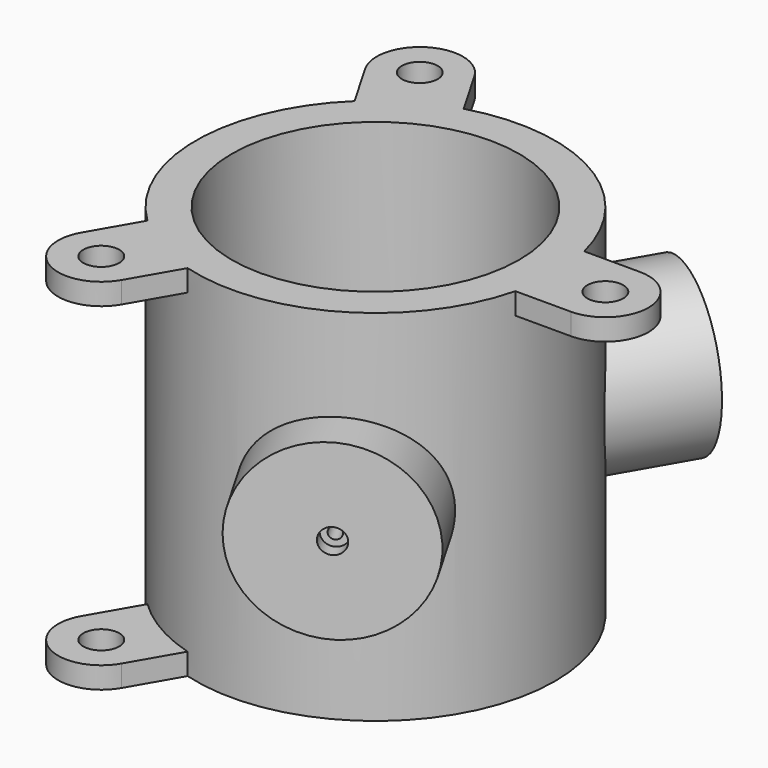
from build123d import *

# Parameters (mm, degrees)
F1_R             = 125
F1_R_2           = 100
F2_DEPTH         = 250
F3_R             = 12.5
F4_DEPTH         = 15
F4_COPIES_COUNT  = 3
F4_COPIES1_COUNT = 2
F10_R            = 56.8493867215
F10_R_2          = 5
F10_R_3          = 28.1619206838
F11_DEPTH        = 68.6754869442
F15_R            = 60.4503373428
F18_D            = 8.5
F18_CBORE_D      = 17.25
F18_CBORE_DEPTH  = 10


# Not quite as in the source:
# - ends of sketch curves that miss each other by under 0.0002 mm in the source are joined
# - a pattern or mirror of a feature is missing from the dataset's text; its kind, count and spacing are read off the source's solid


with BuildPart() as f2:
    # F1 (on offset) → F2 (new body)
    with BuildSketch(Plane.XY.offset(125)):
        Circle(F1_R)
        Circle(F1_R_2, mode=Mode.SUBTRACT)
    extrude(amount=-F2_DEPTH)

    # F3 (on face) → F4 (join)
    with BuildSketch(Plane.XY.offset(125)):
        with BuildLine():
            Line((-105.9807621135, 123.5640646055), (-86.6540676111, 90.0892477849))
            ThreePointArc((-86.6540676111, 90.0892477849), (-62.5, 108.2531754731), (-34.692543384, 120.0892477849))
            Line((-34.692543384, 120.0892477849), (-53.9970505647, 153.5256350369))
            ThreePointArc((-53.9970505647, 153.5256350369), (-54.008151328, 153.5448457136), (-54.0192378865, 153.5640646055))
            ThreePointArc((-54.0192378865, 153.5640646055), (-95, 164.544826719), (-105.9807621135, 123.5640646055))
        make_face()
        with Locations((-80, 138.5640646055)):
            Circle(F3_R, mode=Mode.SUBTRACT)
    f4 = extrude(amount=-F4_DEPTH)

    # F4_copies: F4 ×3 about axis
    f4_copies_axis = Axis((0, 0, 0), (0, 0, 1))
    for i in range(1, F4_COPIES_COUNT):
        add(f4.rotate(f4_copies_axis, i * 360 / F4_COPIES_COUNT))

    # F4_copies1: F4 ×2 about axis
    f4_copies1_axis = Axis((0, 0, 0), (1, 0, 0))
    for i in range(1, F4_COPIES1_COUNT):
        add(f4.rotate(f4_copies1_axis, i * 360 / F4_COPIES1_COUNT))

    # F10 (on offset) → F11 (join, through all)
    with BuildSketch(Plane(origin=(90, 155.8845726812, 0), x_dir=(-0.8660254038, 0.5, 0), z_dir=(0.5, 0.8660254038, 0))):
        Circle(F10_R)
        with Locations((-36.7784088222, -21.2340242338)):
            Circle(F10_R_2, mode=Mode.SUBTRACT)
        with Locations((36.7784088222, -21.2340242338)):
            Circle(F10_R_2, mode=Mode.SUBTRACT)
        Circle(F10_R_3, mode=Mode.SUBTRACT)
        with Locations((0, 42.4680484677)):
            Circle(F10_R_2, mode=Mode.SUBTRACT)
    extrude(amount=-F11_DEPTH)

    # F15 (on offset) → F16 (join, up to the next surface of F2)
    with BuildSketch(Plane(origin=(77.4998450043, -134.2344088806, 0), x_dir=(-0.8660265969, -0.4999979334, 0), z_dir=(-0.4999979334, 0.8660265969, 0))):
        Circle(F15_R)
    extrude(until=Until.NEXT)

    # F18 (through all)
    with Locations(Plane(origin=(77.4998450043, -134.2344088806, 0), x_dir=(0.8660265969, 0.4999979334, 0), z_dir=(0.4999979334, -0.8660265969, 0))):
        with Locations((0, 0)):
            CounterBoreHole(F18_D / 2, F18_CBORE_D / 2, F18_CBORE_DEPTH)


solid = f2.part
